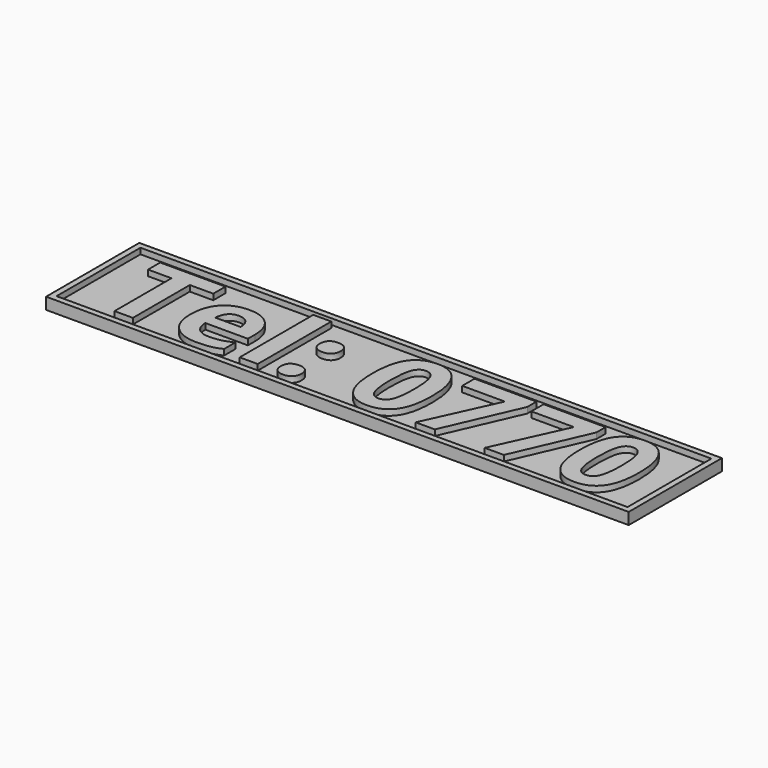
from build123d import *

# Parameters (mm, degrees)
F0_W         = 196
F0_H         = 36
F1_DEPTH     = 2
F0_W_2       = 200
F0_H_2       = 40
F2_DEPTH     = 4
F3_TEXT_SIZE = 41.547949652
F4_DEPTH     = 2


# Not quite as in the source:
# - Text() gives the source's letters only with a copy of the font that has no kerning and outlines rounded to 1/6400 em; it was checked with that copy


with BuildPart() as f1:
    # F0 (on Top) → F1 (new body)
    with BuildSketch(Plane.XY):
        Rectangle(F0_W, F0_H)
    extrude(amount=F1_DEPTH)

    # F0 (on Top) → F2 (join)
    with BuildSketch(Plane.XY):
        Rectangle(F0_W_2, F0_H_2)
        Rectangle(F0_W, F0_H, mode=Mode.SUBTRACT)
    extrude(amount=F2_DEPTH)

    # F3 (on face) → F4 (join)
    with BuildSketch(Plane.XY.offset(2)):
        with Locations((-89.3254178106, -15.0749322411)):
            Text('Tel: 0770', F3_TEXT_SIZE, font='Open Sans', font_style=FontStyle.BOLD, text_align=(TextAlign.LEFT, TextAlign.BOTTOM))
    extrude(amount=F4_DEPTH)


solid = f1.part
